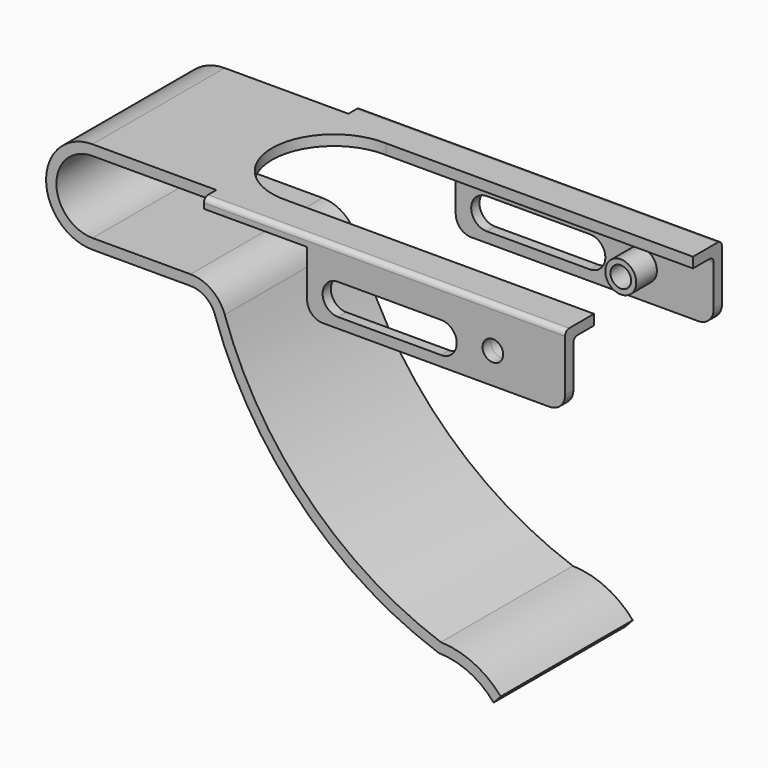
from build123d import *

# Parameters (mm, degrees)
F1_DEPTH  = 16
F2_W      = 70
F2_H      = 3
F3_DEPTH  = 2
F4_W      = 50
F4_H      = 14
F5_DEPTH  = 2
F6_R      = 0.99999
F9_DEPTH  = 2
F11_DEPTH = 38.001
F13_D     = 4
F14_R     = 3
F14_R_2   = 2
F15_DEPTH = 5
F16_R     = 3


# Not quite as in the source:
# - a fillet or chamfer is up to 0.001 mm smaller than in the source, because OpenCascade refuses the exact size
# - a pattern or mirror of a feature is missing from the dataset's text; its kind, count and spacing are read off the source's solid


with BuildPart() as f1:
    # F0 (on Front) → F1 (new body)
    with BuildSketch(Plane.XZ):
        with BuildLine():
            Line((94, 9), (0, 9))
            ThreePointArc((0, 9), (-9, 0), (0, -9))
            Line((0, -9), (19, -9))
            ThreePointArc((19, -9), (21.9107246536, -9.9345748081), (23.7333333333, -12.3889272035))
            ThreePointArc((23.7333333333, -12.3889272035), (40.3930033582, -39.2216179023), (67.1516242057, -56))
            ThreePointArc((67.1516242057, -56), (72.9993471235, -57.3376618382), (77.7503977132, -61))
            Line((77.7503977132, -61), (79.1305544342, -59.4934290732))
            ThreePointArc((79.1305544342, -59.4934290732), (73.8943105869, -55.5314515361), (67.507653226, -54.0062881394))
            ThreePointArc((67.507653226, -54.0062881394), (41.6996239436, -37.699069728), (25.6266664621, -11.7444981545))
            ThreePointArc((25.6266664621, -11.7444981545), (23.0750143892, -8.308404907), (19, -7.0000002161))
            Line((19, -7.0000002161), (0, -7.0000002161))
            ThreePointArc((0, -7.0000002161), (-7.0000002161, 0), (0, 7.0000002161))
            Line((0, 7.0000002161), (94, 7.0000002161))
            Line((94, 7.0000002161), (94, 9))
        make_face()
    extrude(amount=F1_DEPTH)

    # F2 (on face) → F3 (join)
    with BuildSketch(Plane.XY.offset(9)):
        with Locations((59, -17.5)):
            Rectangle(F2_W, F2_H)
    extrude(amount=-F3_DEPTH)

    # F4 (on face) → F5 (join)
    with BuildSketch(Plane.XZ.offset(19)):
        with Locations((69, 2)):
            Rectangle(F4_W, F4_H)
    extrude(amount=-F5_DEPTH)

    # F6 (radius 1 in the source; OpenCascade refuses exactly that, so slightly less here)
    f6_edges = [f1.edges().sort_by_distance(p)[0] for p in [
        (69, -17, 7),
        (59, -19, 9),
    ]]
    fillet(f6_edges, radius=F6_R)

    # F7: F1 across face


with BuildPart() as f1_1:
    add(f1.part)
    add(f1.part.mirror(Plane(origin=(37.3146952464, 0, -11.3167767816), x_dir=(1, 0, 0), z_dir=(0, 1, 0))))

    # F8 (on face) → F9 (cut)
    with BuildSketch(Plane.XY.offset(9)):
        with BuildLine():
            Line((94, 11.9899458001), (34.491120871, 11.9899458001))
            ThreePointArc((34.491120871, 11.9899458001), (22.0000006537, 0.0039610115), (34.4832053788, -11.9902674099))
            Line((34.4832053788, -11.9902674099), (94, -11.9902674099))
            Line((94, -11.9902674099), (94, 11.9899458001))
        make_face()
    extrude(amount=-F9_DEPTH, mode=Mode.SUBTRACT)

    # F10 (on face) → F11 (cut, through all)
    with BuildSketch(Plane.XZ.offset(19)):
        with BuildLine():
            ThreePointArc((50, 3), (47, 0), (50, -3))
            Line((50, -3), (70, -3))
            ThreePointArc((70, -3), (73, 0), (70, 3))
            Line((70, 3), (50, 3))
        make_face()
    extrude(amount=-F11_DEPTH, mode=Mode.SUBTRACT)

    # F13 (through all)
    with Locations(Plane.XZ.offset(19)):
        with Locations((80, 1)):
            Hole(F13_D / 2)

    # F14 (on face) → F15 (join)
    with BuildSketch(Plane(origin=(0, -17, 0), x_dir=(-1, 0, 0), z_dir=(0, 1, 0))):
        with Locations((-80, 1)):
            Circle(F14_R)
        with Locations((-80, 1)):
            Circle(F14_R_2, mode=Mode.SUBTRACT)
    f15 = extrude(amount=F15_DEPTH)

    # F15_copies: F15 across plane
    add(f15.mirror(Plane.ZX))

    # F16
    f16_edges = [f1_1.edges().sort_by_distance(p)[0] for p in [
        (94, 18, -5),
        (94, -18, -5),
        (44, -18, -5),
        (44, 18, -5),
    ]]
    fillet(f16_edges, radius=F16_R)


solid = f1_1.part
